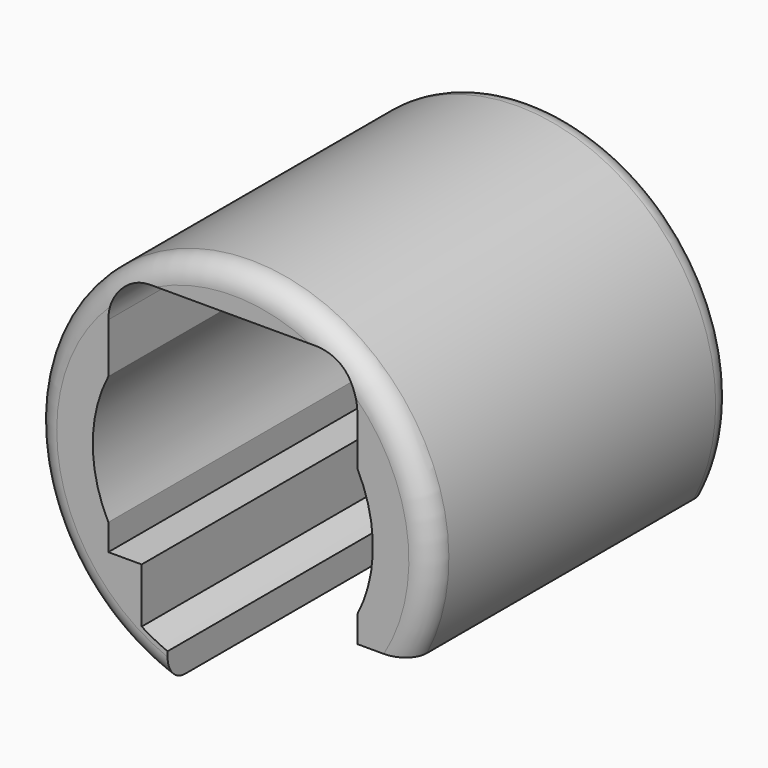
from build123d import *

# Parameters (mm, degrees)
F0_R        = 44.59812
F1_DEPTH    = 85
F3_DEPTH    = 85.001
F4_T2_ANGLE = 310.1787489512
F4_T4_ANGLE = 310.1787489512


# Not quite as in the source:
# - a fillet or chamfer that OpenCascade refuses, or shapes differently, is made with other operations: its cross-section is extruded or revolved along the edge and cut away or added


with BuildPart() as f1:
    # F0 (on Front) → F1 (new body)
    with BuildSketch(Plane.XZ):
        with Locations((20.5, 21.991262728)):
            Circle(F0_R)
        with BuildLine():
            ThreePointArc((62.0981215365, 21.991262728), (57.0788738932, 2.1824338865), (43.2323802204, -12.8461109515))
            ThreePointArc((43.2323802204, -12.8461109515), (-16.0788738932, 41.8000915695), (62.0981215365, 21.991262728))
        make_face(mode=Mode.SUBTRACT)
        with BuildLine():
            ThreePointArc((62.0981215365, 21.991262728), (-16.0788738932, 41.8000915695), (43.2323802204, -12.8461109515))
            ThreePointArc((43.2323802204, -12.8461109515), (57.0788738932, 2.1824338865), (62.0981215365, 21.991262728))
        make_face()
        with BuildLine():
            Line((48.5, 7.5603930383), (48.5, 1.641262728))
            Line((48.5, 1.641262728), (45.5, 1.641262728))
            Line((45.5, 1.641262728), (45.5, -8.658737272))
            ThreePointArc((45.5, -8.658737272), (44.896697687, -11.0397138467), (43.2323802204, -12.8461109515))
            ThreePointArc((43.2323802204, -12.8461109515), (41.9253300675, -13.4512767031), (40.5, -13.658737272))
            Line((40.5, -13.658737272), (5.8251916537, -13.658737272))
            ThreePointArc((5.8251916537, -13.658737272), (2.8487454964, -12.2827174093), (0, -10.658737272))
            Line((0, -10.658737272), (0, 1.641262728))
            Line((0, 1.641262728), (-7.5, 1.641262728))
            Line((-7.5, 1.641262728), (-7.5, 7.5603930383))
            ThreePointArc((-7.5, 7.5603930383), (-11, 21.991262728), (-7.5, 36.4221324176))
            Line((-7.5, 36.4221324176), (-7.5, 40.641262728))
            Line((-7.5, 40.641262728), (-7.5, 45.641262728))
            Line((-7.5, 45.641262728), (-7.5, 47.641262728))
            ThreePointArc((-7.5, 47.641262728), (-4.5710678119, 54.7123305398), (2.5, 57.641262728))
            Line((2.5, 57.641262728), (38.5, 57.641262728))
            ThreePointArc((38.5, 57.641262728), (45.5710678119, 54.7123305398), (48.5, 47.641262728))
            Line((48.5, 47.641262728), (48.5, 45.641262728))
            Line((48.5, 45.641262728), (48.5, 40.641262728))
            Line((48.5, 40.641262728), (48.5, 36.4221324176))
            ThreePointArc((48.5, 36.4221324176), (52, 21.991262728), (48.5, 7.5603930383))
        make_face(mode=Mode.SUBTRACT)
    extrude(amount=F1_DEPTH)

    # F2 (on face) → F3 (cut, through all)
    with BuildSketch(Plane.XZ.offset(85)):
        with BuildLine():
            Line((5.8251916537, -13.658737272), (5.8251916537, -20.1233702104))
            ThreePointArc((5.8251916537, -20.1233702104), (37.0770201947, -19.4115718247), (60.1846293612, 1.641262728))
            Line((60.1846293612, 1.641262728), (48.5, 1.641262728))
            Line((48.5, 1.641262728), (45.5, 1.641262728))
            Line((45.5, 1.641262728), (45.5, -8.658737272))
            ThreePointArc((45.5, -8.658737272), (44.0355339059, -12.194271178), (40.5, -13.658737272))
            Line((40.5, -13.658737272), (5.8251916537, -13.658737272))
        make_face()
    extrude(amount=-F3_DEPTH, mode=Mode.SUBTRACT)

    # F4: fillet of radius 5 on 2 edges, made by hand

    # F4_s1 → F4_t2 (revolve, cut)
    with BuildSketch(Plane(origin=(20.6066088897, 0, 21.8909083866), x_dir=(0, 1, 0), z_dir=(-0.6854246842, 0, -0.7281435314))):
        with BuildLine():
            ThreePointArc((-85, 39.4517080838), (-83.5355339059, 42.9872419898), (-80, 44.4517080838))
            Line((-80, 44.4517080838), (-85, 44.4517080838))
            Line((-85, 44.4517080838), (-85, 39.4517080838))
        make_face()
    revolve(axis=Axis((20.5, -85, 21.991262728), (0, -1, 0)), revolution_arc=F4_T2_ANGLE, mode=Mode.SUBTRACT)

    # F4_s3 → F4_t4 (revolve, cut)
    with BuildSketch(Plane(origin=(19.2566159931, 0, -1.0396200852), x_dir=(0, 1, 0), z_dir=(0.998545843, 0, -0.0539091767))):
        with BuildLine():
            ThreePointArc((-5, -21.533697897), (-1.4644660941, -20.0692318029), (0, -16.533697897))
            Line((0, -16.533697897), (0, -21.533697897))
            Line((0, -21.533697897), (-5, -21.533697897))
        make_face()
    revolve(axis=Axis((20.5, 0, 21.991262728), (0, 1, 0)), revolution_arc=F4_T4_ANGLE, mode=Mode.SUBTRACT)


solid = f1.part
